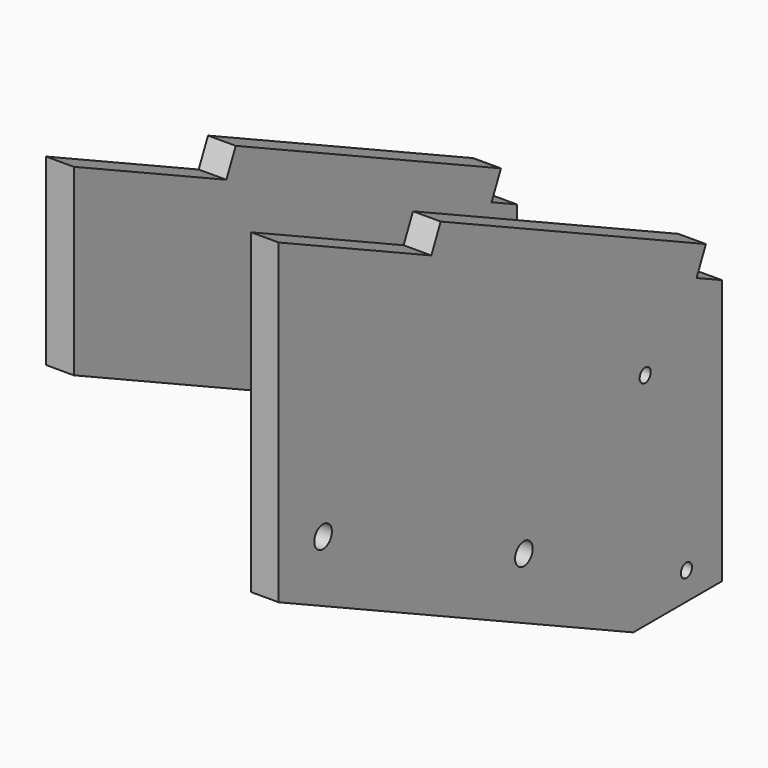
from build123d import *

# Parameters (mm, degrees)
F0_R       = 1.5875
F1_DEPTH   = 6.35
F3_DEPTH   = 46.99
F4_R       = 1.5875
F5_DEPTH   = 6.35
F6_W       = 3.81
F6_H       = 76.2
F7_DEPTH   = 6.35
F8_R       = 2.5273
F9_DEPTH   = 6.35
F10_W      = 6.35
F10_H      = 5.0546
F10_H_2    = 51.2035957082
F11_DEPTH  = 6.35
F11_FACE_W = 6.35
F11_FACE_H = 6.35
F12_DEPTH  = 28.6456124865


with BuildPart() as f1:
    # F0 (on Right) → F1 (new body)
    with BuildSketch(Plane.YZ):
        Polygon((63.5, -63.5), (63.5, 4.2789274143), (-63.5, 63.5), (-63.5, -16.1231419315), (38.1, -63.5), align=None)
        with Locations((53.34, -57.15)):
            Circle(F0_R, mode=Mode.SUBTRACT)
        with Locations((41.5067932579, -12.9878712221)):
            Circle(F0_R, mode=Mode.SUBTRACT)
    extrude(amount=F1_DEPTH)

    # F8 (on face) → F9 (cut, through all)
    with BuildSketch(Plane.YZ.offset(6.35)):
        with Locations((-50.8, -8.0323496192)):
            Circle(F8_R)
        with Locations((6.7505444768, -34.8686092397)):
            Circle(F8_R)
    extrude(amount=-F9_DEPTH, mode=Mode.SUBTRACT)


with BuildPart() as f3:
    # F2 (on face) → F3 (new body)
    with BuildSketch(Plane(origin=(0, 0, 0), x_dir=(0, -1, 0), z_dir=(-1, 0, 0))):
        Polygon((11.7045099709, 32.3409165561), (63.5, 56.4935502146), (63.5, 63.5), (9.0208840088, 38.0959710038), align=None)
        Polygon((-63.5, -2.7275223711), (-55.0613195903, 1.2074989287), (-57.7449455523, 6.9625533764), (-63.5, 4.2789274143), align=None)
        Polygon((-55.0613195903, 1.2074989287), (11.7045099709, 32.3409165561), (9.0208840088, 38.0959710038), (-57.7449455523, 6.9625533764), align=None)
    extrude(amount=F3_DEPTH)

    # F4 (on face) → F5 (join)
    with BuildSketch(Plane(origin=(-46.99, 0, 0), x_dir=(0, -1, 0), z_dir=(-1, 0, 0))):
        Polygon((63.5, 63.5), (-63.5, 4.2789274143), (-63.5, -21.1210725857), (-12.7, -21.1210725857), (63.5, 14.4115709657), align=None)
        with Locations((-41.5067932579, -12.9878712221)):
            Circle(F4_R, mode=Mode.SUBTRACT)
    extrude(amount=-F5_DEPTH)

    # F6 (on face) → F7 (cut, through all)
    with BuildSketch(Plane(origin=(0, 12.9804176766, 27.8365955385), x_dir=(1, 0, 0), z_dir=(0, 0.4226182617, 0.906307787))):
        with Locations((-1.905, 11.2921916109)):
            Rectangle(F6_W, F6_H)
        with Locations((-38.735, 11.2921916109)):
            Rectangle(F6_W, F6_H)
    extrude(amount=-F7_DEPTH, mode=Mode.SUBTRACT)


with BuildPart() as f11_tool:
    # F10 (on face) → F11 (new body)
    with BuildSketch(Plane(origin=(0, 12.9804176766, 27.8365955385), x_dir=(1, 0, 0), z_dir=(0, 0.4226182617, 0.906307787))):
        Polygon((-3.81, 49.3921916109), (0, 49.3921916109), (0, 50.6875916109), (0, 55.7421916109), (-46.99, 55.7421916109), (-46.99, 50.6875916109), (-40.64, 50.6875916109), (-40.64, 49.3921916109), (-36.83, 49.3921916109), (-36.83, -26.8078083891), (-40.64, -26.8078083891), (-40.64, -33.1832083891), (-46.99, -33.1832083891), (-46.99, -84.3868040974), (0, -84.3868040974), (0, -33.1832083891), (0, -26.8078083891), (-3.81, -26.8078083891), align=None)
        with Locations((3.175, 53.2148916109)):
            Rectangle(F10_W, F10_H)
        with Locations((3.175, -58.7850062432)):
            Rectangle(F10_W, F10_H_2)
    extrude(amount=-F11_DEPTH)


with BuildPart() as f1_1:
    add(f1.part)

    # F11: cut by f11_tool
    add(f11_tool.part, mode=Mode.SUBTRACT)


with BuildPart() as f3_1:
    add(f3.part)

    # F11: cut by f11_tool
    add(f11_tool.part, mode=Mode.SUBTRACT)


with BuildPart() as f12_tool:
    # F11_face (on face) + F11_face1 (on face) → F12 (new body, through all)
    with BuildSketch(Plane(origin=(3.175, 62.158187019, 1.4014001905), x_dir=(1, 0, 0), z_dir=(0, -0.906307787, 0.4226182617))):
        Rectangle(F11_FACE_W, F11_FACE_H)
    with BuildSketch(Plane(origin=(-23.495, 62.158187019, 1.4014001905), x_dir=(1, 0, 0), z_dir=(0, -0.906307787, 0.4226182617))):
        Polygon((23.495, 3.175), (-23.495, 3.175), (-23.495, -3.175), (-17.145, -3.175), (23.495, -3.175), align=None)
    extrude(amount=-F12_DEPTH)


with BuildPart() as f1_2:
    add(f1_1.part)

    # F12: cut by f12_tool
    add(f12_tool.part, mode=Mode.SUBTRACT)


with BuildPart() as f3_2:
    add(f3_1.part)

    # F12: cut by f12_tool
    add(f12_tool.part, mode=Mode.SUBTRACT)


solid = Compound([f1_2.part, f3_2.part])
